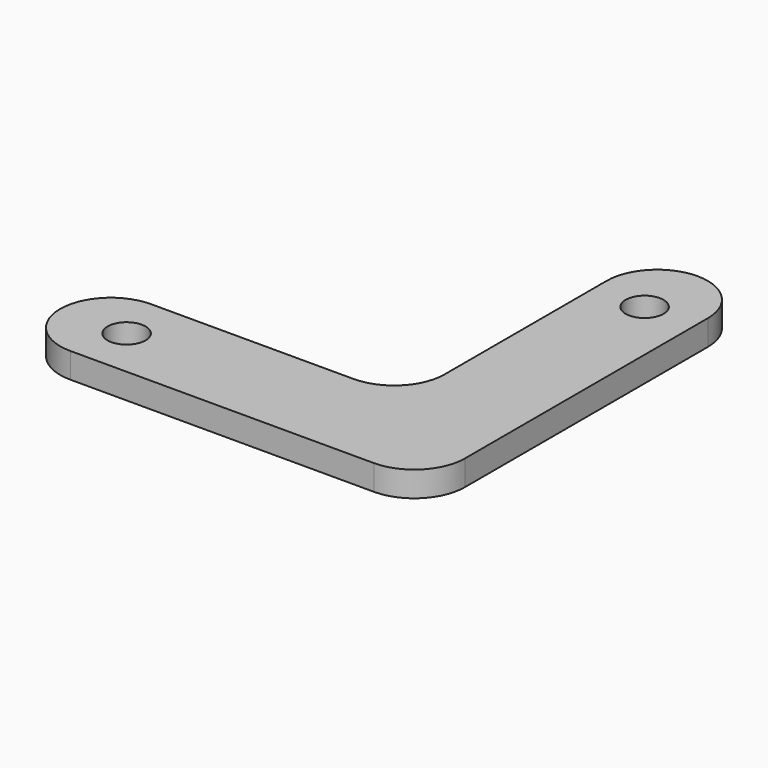
from build123d import *

# Parameters (mm, degrees)
F0_R     = 2.38125
F1_DEPTH = 3.175
F2_R     = 6.34999


# Not quite as in the source:
# - a fillet or chamfer is up to 0.001 mm smaller than in the source, because OpenCascade refuses the exact size


with BuildPart() as f1:
    # F0 (on Top) → F1 (new body)
    with BuildSketch(Plane.XY):
        Polygon((0, 12.7), (0, 0), (50.8, 0), (50.8, 50.8), (38.1, 50.8), (38.1, 12.7), align=None)
        with Locations((8.3286329803, 6.35)):
            Circle(F0_R, mode=Mode.SUBTRACT)
        with Locations((44.45, 42.4713670197)):
            Circle(F0_R, mode=Mode.SUBTRACT)
    extrude(amount=F1_DEPTH)

    # F2 (radius 6.35 in the source; OpenCascade refuses exactly that, so slightly less here)
    f2_edges = [f1.edges().sort_by_distance(p)[0] for p in [
        (0, 0, 1.5875),
        (0, 12.7, 1.5875),
        (38.1, 50.8, 1.5875),
        (38.1, 12.7, 1.5875),
        (50.8, 0, 1.5875),
        (50.8, 50.8, 1.5875),
    ]]
    fillet(f2_edges, radius=F2_R)


solid = f1.part
